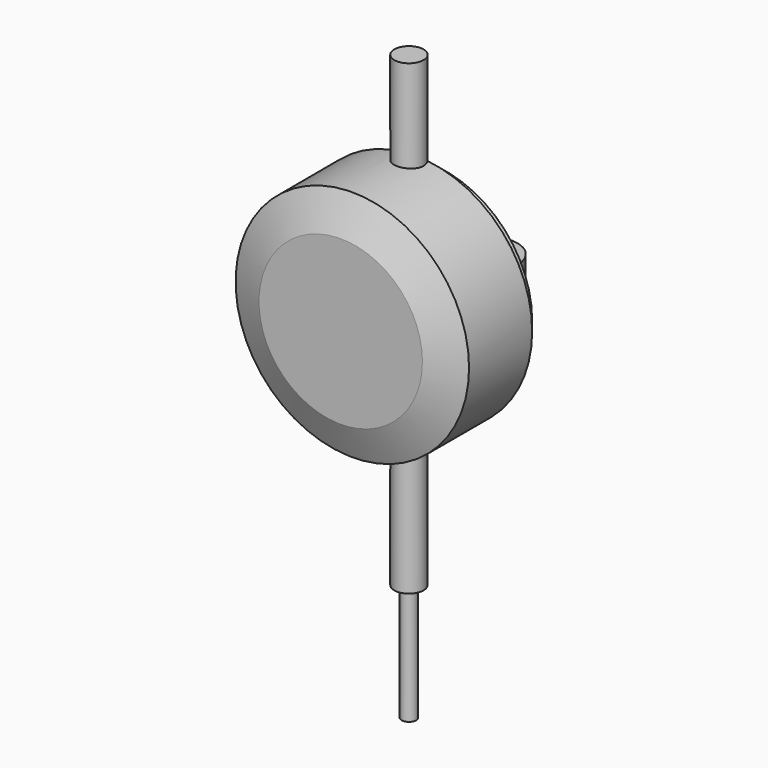
from build123d import *

# Parameters (mm, degrees)
F0_R          = 3.175
F1_DEPTH      = 6.477
F2_R          = 22.86
F2_W          = 19.05
F2_H          = 6.477
F3_DEPTH      = 3.175
F4_R          = 25.4
F4_R_2        = 22.86
F4_W          = 19.05
F4_H          = 6.477
F5_DEPTH      = 20.32
F6_SIZE       = 2.54
F8_R          = 3.175
F9_DEPTH      = 50.8
F9_DEPTH_BACK = 50.8
F10_R         = 1.5875
F11_DEPTH     = 25.4


# Not quite as in the source:
# - a fillet or chamfer that OpenCascade refuses, or shapes differently, is made with other operations: its cross-section is extruded or revolved along the edge and cut away or added


with BuildPart() as f1:
    # F0 (on Top) → F1 (new body)
    with BuildSketch(Plane.XY):
        with BuildLine():
            ThreePointArc((9.525, 3.175), (7.6651280605, 7.6651280605), (3.175, 9.525))
            Line((3.175, 9.525), (-3.175, 9.525))
            ThreePointArc((-3.175, 9.525), (-7.6651280605, 7.6651280605), (-9.525, 3.175))
            Line((-9.525, 3.175), (-9.525, -9.525))
            Line((-9.525, -9.525), (9.525, -9.525))
            Line((9.525, -9.525), (9.525, 3.175))
        make_face()
        Circle(F0_R, mode=Mode.SUBTRACT)
    extrude(amount=F1_DEPTH)


with BuildPart() as f3:
    # F2 (on face) → F3 (new body)
    with BuildSketch(Plane.XZ.offset(9.525)):
        with Locations((0, 5.3216813781)):
            Circle(F2_R)
        with Locations((0, 3.2385)):
            Rectangle(F2_W, F2_H, mode=Mode.SUBTRACT)
    extrude(amount=F3_DEPTH)

    # F4 (on face) → F5 (join)
    with BuildSketch(Plane.XZ.offset(12.7)):
        with Locations((0, 5.3216813781)):
            Circle(F4_R)
        with Locations((0, 5.3216813781)):
            Circle(F4_R_2, mode=Mode.SUBTRACT)
        with Locations((0, 5.3216813781)):
            Circle(F4_R_2)
        with Locations((0, 3.2385)):
            Rectangle(F4_W, F4_H, mode=Mode.SUBTRACT)
        with Locations((0, 3.2385)):
            Rectangle(F4_W, F4_H)
    extrude(amount=F5_DEPTH)

    # F6
    f6_edges = [f3.edges().sort_by_distance(p)[0] for p in [
        (-25.4, -33.02, 5.321681),
    ]]
    chamfer(f6_edges, length=F6_SIZE)

    # F7: chamfer of 5.08 on 1 edges, made by hand

    # F7_s1 → F7_t2 (revolve, cut)
    with BuildSketch(Plane.XY.offset(5.3216813781)):
        Polygon((26.4521024484, -29.4278975516), (17.78, -33.02), (22.86, -33.02), align=None)
    revolve(axis=Axis((0, -33.02, 5.3216813781), (0, -1, 0)), mode=Mode.SUBTRACT)

    # F8 (on Top) → F9 (join, two sides)
    with BuildSketch(Plane.XY) as f9_sk:
        with Locations((0, -14.4734445528)):
            Circle(F8_R)
    extrude(amount=F9_DEPTH)
    extrude(f9_sk.sketch, amount=-F9_DEPTH_BACK)

    # F10 (on face) → F11 (join)
    with BuildSketch(Plane(origin=(0, 0, -50.8), x_dir=(1, 0, 0), z_dir=(0, 0, -1))):
        with Locations((0, 14.4734445528)):
            Circle(F10_R)
    extrude(amount=F11_DEPTH)


solid = Compound([f1.part, f3.part])
